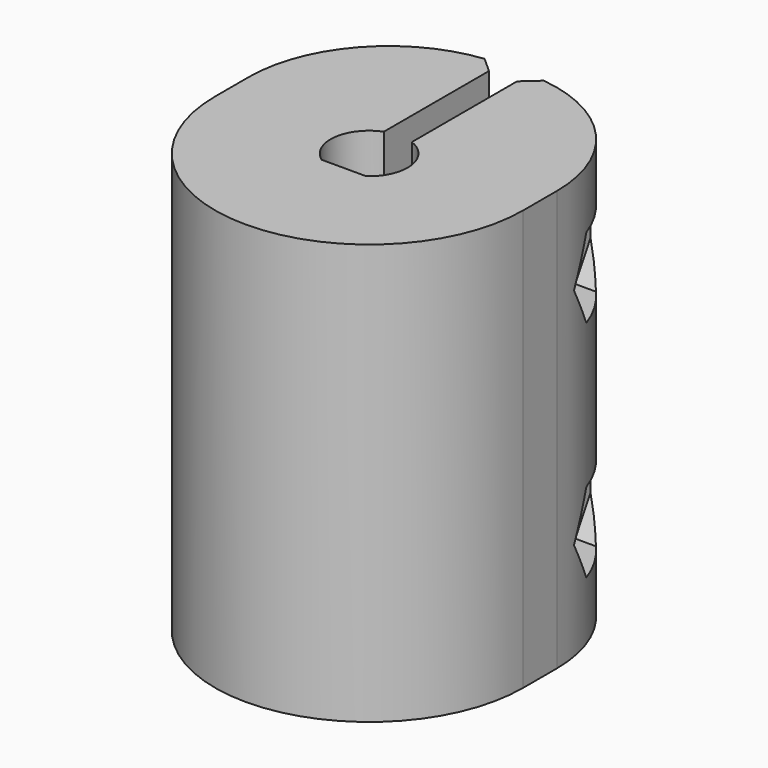
from build123d import *

# Parameters (mm, degrees)
F0_R         = 5.25
F1_DEPTH     = 30
F2_DEPTH     = 15
F3_DEPTH     = 30
F4_R         = 2
F6_DEPTH     = 22
F4_R_2       = 3.5
F7_DEPTH     = 4
F5_R         = 2
F8_DEPTH     = 4
F9_W         = 1
F9_H         = 30
F10_DEPTH    = 15
F11_T1_DEPTH = 80
F12_T1_DEPTH = 35.7073493424


# Not quite as in the source:
# - a fillet or chamfer that OpenCascade refuses, or shapes differently, is made with other operations: its cross-section is extruded or revolved along the edge and cut away or added


with BuildPart() as f1:
    # F0 (on Top) → F1 (new body)
    with BuildSketch(Plane.XY):
        with BuildLine():
            ThreePointArc((-11, 0), (0, -11), (11, 0))
            ThreePointArc((11, 0), (7.7781745931, 7.7781745931), (0, 11))
            ThreePointArc((0, 11), (-7.7781745931, 7.7781745931), (-11, 0))
        make_face()
        Circle(F0_R, mode=Mode.SUBTRACT)
        Circle(F0_R)
        with BuildLine():
            ThreePointArc((-1.5811388301, -2.25), (-1.2677476518, 2.4403515918), (2.75, 0))
            ThreePointArc((2.75, 0), (2.4403515918, -1.2677476518), (1.5811388301, -2.25))
            ThreePointArc((1.5811388301, -2.25), (0, -2.75), (-1.5811388301, -2.25))
        make_face(mode=Mode.SUBTRACT)
        with BuildLine():
            ThreePointArc((-11, 0), (-7.7781745931, 7.7781745931), (0, 11))
            Line((0, 11), (-11, 11))
            Line((-11, 11), (-11, 0))
        make_face()
        with BuildLine():
            ThreePointArc((0, 11), (7.7781745931, 7.7781745931), (11, 0))
            Line((11, 0), (11, 11))
            Line((11, 11), (0, 11))
        make_face()
        Polygon((-11, 11), (0, 11), (11, 11), (11, 13), (-11, 13), align=None)
        with BuildLine():
            Line((0, -2.25), (-1.5811388301, -2.25))
            ThreePointArc((-1.5811388301, -2.25), (0, -2.75), (1.5811388301, -2.25))
            Line((1.5811388301, -2.25), (0, -2.25))
        make_face()
        with BuildLine():
            ThreePointArc((1.5811388301, -2.25), (2.4403515918, -1.2677476518), (2.75, 0))
            ThreePointArc((2.75, 0), (-1.2677476518, 2.4403515918), (-1.5811388301, -2.25))
            Line((-1.5811388301, -2.25), (0, -2.25))
            Line((0, -2.25), (1.5811388301, -2.25))
        make_face()
    extrude(amount=F1_DEPTH)

    # F0 (on Top) → F2 (cut)
    with BuildSketch(Plane.XY):
        Circle(F0_R)
        with BuildLine():
            ThreePointArc((-1.5811388301, -2.25), (-1.2677476518, 2.4403515918), (2.75, 0))
            ThreePointArc((2.75, 0), (2.4403515918, -1.2677476518), (1.5811388301, -2.25))
            ThreePointArc((1.5811388301, -2.25), (0, -2.75), (-1.5811388301, -2.25))
        make_face(mode=Mode.SUBTRACT)
        with BuildLine():
            Line((0, -2.25), (-1.5811388301, -2.25))
            ThreePointArc((-1.5811388301, -2.25), (0, -2.75), (1.5811388301, -2.25))
            Line((1.5811388301, -2.25), (0, -2.25))
        make_face()
    extrude(amount=F2_DEPTH, mode=Mode.SUBTRACT)

    # F0 (on Top) → F3 (cut)
    with BuildSketch(Plane.XY):
        with BuildLine():
            ThreePointArc((1.5811388301, -2.25), (2.4403515918, -1.2677476518), (2.75, 0))
            ThreePointArc((2.75, 0), (-1.2677476518, 2.4403515918), (-1.5811388301, -2.25))
            Line((-1.5811388301, -2.25), (0, -2.25))
            Line((0, -2.25), (1.5811388301, -2.25))
        make_face()
    extrude(amount=F3_DEPTH, mode=Mode.SUBTRACT)

    # F4 (on face) → F6 (cut)
    with BuildSketch(Plane(origin=(-11, 0, 0), x_dir=(0, -1, 0), z_dir=(-1, 0, 0))):
        with Locations((-8, 7)):
            Circle(F4_R)
        with Locations((-8, 23)):
            Circle(F4_R)
    extrude(amount=-F6_DEPTH, mode=Mode.SUBTRACT)

    # F4 (on face) → F7 (cut)
    with BuildSketch(Plane(origin=(-11, 0, 0), x_dir=(0, -1, 0), z_dir=(-1, 0, 0))):
        with Locations((-8, 7)):
            Circle(F4_R_2)
        with Locations((-8, 7)):
            Circle(F4_R, mode=Mode.SUBTRACT)
        with Locations((-8, 23)):
            Circle(F4_R_2)
        with Locations((-8, 23)):
            Circle(F4_R, mode=Mode.SUBTRACT)
    extrude(amount=-F7_DEPTH, mode=Mode.SUBTRACT)

    # F5 (on face) → F8 (cut)
    with BuildSketch(Plane.YZ.offset(11)):
        Polygon((6.3545517328, 4.15), (9.6454482672, 4.15), (11.2908965344, 7), (9.6454482672, 9.85), (6.3545517328, 9.85), (4.7091034656, 7), align=None)
        with Locations((8, 7)):
            Circle(F5_R, mode=Mode.SUBTRACT)
        Polygon((6.3545517328, 20.15), (9.6454482672, 20.15), (11.2908965344, 23), (9.6454482672, 25.85), (6.3545517328, 25.85), (4.7091034656, 23), align=None)
        with Locations((8, 23)):
            Circle(F5_R, mode=Mode.SUBTRACT)
    extrude(amount=-F8_DEPTH, mode=Mode.SUBTRACT)

    # F9 (on face) → F10 (cut)
    with BuildSketch(Plane(origin=(0, 13, 0), x_dir=(-1, 0, 0), z_dir=(0, 1, 0))):
        with Locations((0.5, 15)):
            Rectangle(F9_W, F9_H)
        with Locations((-0.5, 15)):
            Rectangle(F9_W, F9_H)
    extrude(amount=-F10_DEPTH, mode=Mode.SUBTRACT)

    # F11: fillet of radius 10 on 2 edges, made by hand

    # F11_s2 → F11_t1 (cut)
    with BuildSketch(Plane.XY.offset(-25)):
        with BuildLine():
            ThreePointArc((-1, 13), (-8.0710678119, 10.0710678119), (-11, 3))
            Line((-11, 3), (-11, 13))
            Line((-11, 13), (-1, 13))
        make_face()
        with BuildLine():
            ThreePointArc((1, 13), (8.0710678119, 10.0710678119), (11, 3))
            Line((11, 3), (11, 13))
            Line((11, 13), (1, 13))
        make_face()
    extrude(amount=F11_T1_DEPTH, mode=Mode.SUBTRACT)

    # F12: chamfer of 1 on 2 edges, made by hand

    # F12_s2 → F12_t1 (cut)
    with BuildSketch(Plane.XY.offset(-2.8536746712)):
        with BuildLine():
            Line((-1, 11.94427191), (-2.1111111111, 12.9380799))
            ThreePointArc((-2.1111111111, 12.9380799), (-1.5705391213, 12.983710989), (-1, 13))
            Line((-1, 13), (-1, 11.94427191))
        make_face()
        with BuildLine():
            Line((2.1111111111, 12.9380799), (1, 11.94427191))
            Line((1, 11.94427191), (1, 13))
            ThreePointArc((1, 13), (1.5705391213, 12.983710989), (2.1111111111, 12.9380799))
        make_face()
    extrude(amount=F12_T1_DEPTH, mode=Mode.SUBTRACT)


solid = f1.part
